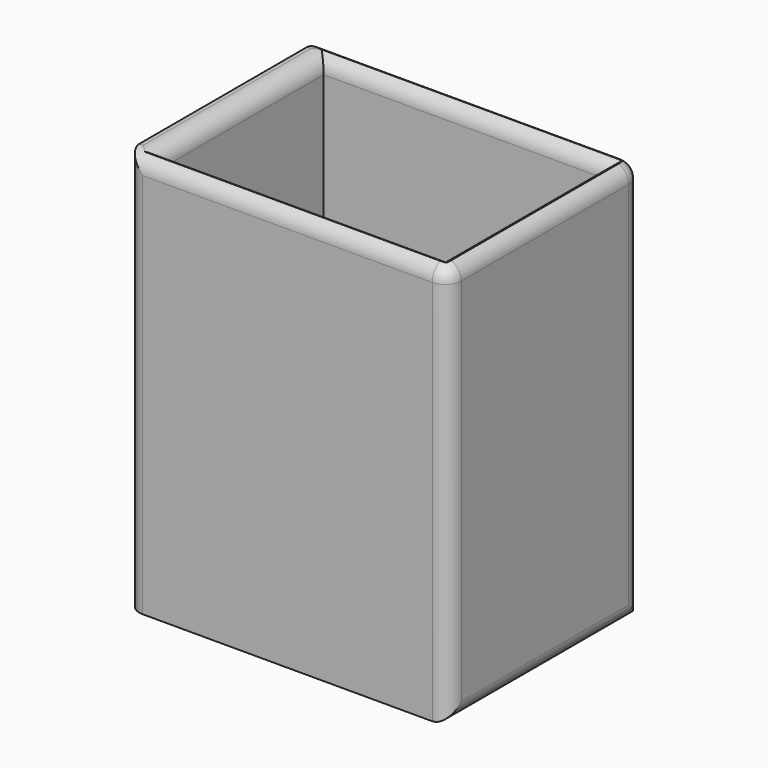
from build123d import *

# Parameters (mm, degrees)
F0_W         = 101.6
F0_H         = 76.2
F1_DEPTH     = 127
F2_T         = -6.35
F3_T1_DEPTH  = 152.4
F3_T3_DEPTH  = 134.62
F3_T5_DEPTH  = 101.6
F3_T7_DEPTH  = 66.04
F3_T9_DEPTH  = 109.22
F3_T11_DEPTH = 88.9
F3_T13_DEPTH = 63.5
F3_S17_W     = 5.1816
F3_S17_H     = 5.1816
F3_T18_DEPTH = 5.1816
F3_S23_W     = 5.1816
F3_S23_H     = 5.1816
F3_T24_DEPTH = 5.1816
F3_T31_DEPTH = 101.6
F3_T36_DEPTH = 76.2
F3_T44_DEPTH = 76.2
F3_T49_DEPTH = 101.6
F3_T57_DEPTH = 101.6
F3_T62_DEPTH = 76.2
F3_T70_DEPTH = 101.6
F3_T75_DEPTH = 76.2


# Not quite as in the source:
# - a fillet or chamfer that OpenCascade refuses, or shapes differently, is made with other operations: its cross-section is extruded or revolved along the edge and cut away or added


with BuildPart() as f1:
    # F0 (on Top) → F1 (new body)
    with BuildSketch(Plane.XY):
        with Locations((74.7453766656, -13.2239237391)):
            Rectangle(F0_W, F0_H)
    extrude(amount=F1_DEPTH)

    # F2
    f2_openings = [f1.faces().sort_by_distance(p)[0] for p in [
        (74.745377, -13.223924, 127),
    ]]
    offset(amount=F2_T, openings=f2_openings)

    # F3: fillet of radius 5.08 on 12 edges, made by hand

    # F3_s2 → F3_t1 (cut)
    with BuildSketch(Plane.XY.offset(-12.7)):
        with BuildLine():
            ThreePointArc((29.0253766656, 24.8760762609), (25.4332742171, 23.3881787093), (23.9453766656, 19.7960762609))
            Line((23.9453766656, 19.7960762609), (23.9453766656, 24.8760762609))
            Line((23.9453766656, 24.8760762609), (29.0253766656, 24.8760762609))
        make_face()
        with BuildLine():
            ThreePointArc((29.0253766656, -51.3239237391), (25.4332742171, -49.8360261876), (23.9453766656, -46.2439237391))
            Line((23.9453766656, -46.2439237391), (23.9453766656, -51.3239237391))
            Line((23.9453766656, -51.3239237391), (29.0253766656, -51.3239237391))
        make_face()
    extrude(amount=F3_T1_DEPTH, mode=Mode.SUBTRACT)

    # F3_s4 → F3_t3 (cut)
    with BuildSketch(Plane.XY.offset(-12.7)):
        with BuildLine():
            ThreePointArc((125.5453766656, 19.7960762609), (124.057479114, 23.3881787093), (120.4653766656, 24.8760762609))
            Line((120.4653766656, 24.8760762609), (125.5453766656, 24.8760762609))
            Line((125.5453766656, 24.8760762609), (125.5453766656, 19.7960762609))
        make_face()
        with BuildLine():
            ThreePointArc((120.4653766656, -51.3239237391), (124.057479114, -49.8360261876), (125.5453766656, -46.2439237391))
            Line((125.5453766656, -46.2439237391), (125.5453766656, -51.3239237391))
            Line((125.5453766656, -51.3239237391), (120.4653766656, -51.3239237391))
        make_face()
    extrude(amount=F3_T3_DEPTH, mode=Mode.SUBTRACT)

    # F3_s6 → F3_t5 (cut)
    with BuildSketch(Plane.XZ.offset(-37.5760762609)):
        with BuildLine():
            ThreePointArc((125.5453766656, 5.08), (124.057479114, 1.4878975516), (120.4653766656, 0))
            Line((120.4653766656, 0), (125.5453766656, 0))
            Line((125.5453766656, 0), (125.5453766656, 5.08))
        make_face()
    extrude(amount=F3_T5_DEPTH, mode=Mode.SUBTRACT)

    # F3_s8 → F3_t7 (cut)
    with BuildSketch(Plane.XZ.offset(-19.7960762609)):
        with BuildLine():
            ThreePointArc((125.5453766656, 121.92), (124.057479114, 125.5121024484), (120.4653766656, 127))
            Line((120.4653766656, 127), (125.5453766656, 127))
            Line((125.5453766656, 127), (125.5453766656, 121.92))
        make_face()
    extrude(amount=F3_T7_DEPTH, mode=Mode.SUBTRACT)

    # F3_s10 → F3_t9 (cut)
    with BuildSketch(Plane.YZ.offset(11.2453766656)):
        with BuildLine():
            ThreePointArc((-51.3239237391, 121.92), (-49.8360261876, 125.5121024484), (-46.2439237391, 127))
            Line((-46.2439237391, 127), (-51.3239237391, 127))
            Line((-51.3239237391, 127), (-51.3239237391, 121.92))
        make_face()
        with BuildLine():
            ThreePointArc((24.8760762609, 121.92), (23.3881787093, 125.5121024484), (19.7960762609, 127))
            Line((19.7960762609, 127), (24.8760762609, 127))
            Line((24.8760762609, 127), (24.8760762609, 121.92))
        make_face()
    extrude(amount=F3_T9_DEPTH, mode=Mode.SUBTRACT)

    # F3_s12 → F3_t11 (cut)
    with BuildSketch(Plane.YZ.offset(30.2953766656)):
        with BuildLine():
            ThreePointArc((23.6060762609, 127), (20.0139738124, 125.5121024484), (18.5260762609, 121.92))
            Line((18.5260762609, 121.92), (18.5260762609, 127))
            Line((18.5260762609, 127), (23.6060762609, 127))
        make_face()
        with BuildLine():
            ThreePointArc((-50.0539237391, 127), (-46.4618212907, 125.5121024484), (-44.9739237391, 121.92))
            Line((-44.9739237391, 121.92), (-44.9739237391, 127))
            Line((-44.9739237391, 127), (-50.0539237391, 127))
        make_face()
    extrude(amount=F3_T11_DEPTH, mode=Mode.SUBTRACT)

    # F3_s14 → F3_t13 (cut)
    with BuildSketch(Plane.XZ.offset(-18.5260762609)):
        with BuildLine():
            ThreePointArc((25.2153766656, 127), (28.807479114, 125.5121024484), (30.2953766656, 121.92))
            Line((30.2953766656, 121.92), (30.2953766656, 127))
            Line((30.2953766656, 127), (25.2153766656, 127))
        make_face()
        with BuildLine():
            ThreePointArc((124.2753766656, 127), (120.6832742171, 125.5121024484), (119.1953766656, 121.92))
            Line((119.1953766656, 121.92), (119.1953766656, 127))
            Line((119.1953766656, 127), (124.2753766656, 127))
        make_face()
    extrude(amount=F3_T13_DEPTH, mode=Mode.SUBTRACT)


with BuildPart() as f3_tool16:
    # F3_s17 → F3_t18 (new body)
    with BuildSketch(Plane.YZ.offset(120.4653766656)):
        with Locations((22.3868762609, 124.5108)):
            Rectangle(F3_S17_W, F3_S17_H)
    extrude(amount=F3_T18_DEPTH)

    # F3_s19 → F3_t20 (revolve, cut)
    with BuildSketch(Plane(origin=(120.4653766656, 19.7960762609, 121.92), x_dir=(0, -0.7071067812, -0.7071067812), z_dir=(0, -0.7071067812, 0.7071067812))):
        with BuildLine():
            ThreePointArc((0, -5.08), (5.08, 0), (0, 5.08))
            Line((0, 5.08), (0, -5.08))
        make_face()
    revolve(axis=Axis((120.4653766656, 19.7960762609, 121.92), (1, 0, 0)), mode=Mode.SUBTRACT)


with BuildPart() as f1_1:
    add(f1.part)

    # F3_t15: cut F3_tool16
    add(f3_tool16.part, mode=Mode.SUBTRACT)


with BuildPart() as f3_tool22:
    # F3_s23 → F3_t24 (new body)
    with BuildSketch(Plane.XZ.offset(46.2439237391)):
        with Locations((123.0561766656, 124.5108)):
            Rectangle(F3_S23_W, F3_S23_H)
    extrude(amount=F3_T24_DEPTH)

    # F3_s25 → F3_t26 (revolve, cut)
    with BuildSketch(Plane(origin=(120.4653766656, -46.2439237391, 121.92), x_dir=(-0.7071067812, 0, -0.7071067812), z_dir=(-0.7071067812, 0, 0.7071067812))):
        with BuildLine():
            ThreePointArc((0, -5.08), (5.08, 0), (0, 5.08))
            Line((0, 5.08), (0, -5.08))
        make_face()
    revolve(axis=Axis((120.4653766656, -46.2439237391, 121.92), (0, -1, 0)), mode=Mode.SUBTRACT)


with BuildPart() as f1_2:
    add(f1_1.part)

    # F3_t21: cut F3_tool22
    add(f3_tool22.part, mode=Mode.SUBTRACT)


with BuildPart() as f3_tool29:
    # F3_s30 → F3_t31 (new body)
    with BuildSketch(Plane.YZ.offset(131.8953766656)):
        with BuildLine():
            ThreePointArc((23.6060762609, 127), (20.0139738124, 125.5121024484), (18.5260762609, 121.92))
            Line((18.5260762609, 121.92), (18.5260762609, 127))
            Line((18.5260762609, 127), (23.6060762609, 127))
        make_face()
    extrude(amount=-F3_T31_DEPTH)

    split(bisect_by=Plane.YZ.offset(125.5453766656), keep=Keep.BOTTOM)

    split(bisect_by=Plane.YZ.offset(119.1953766656), keep=Keep.TOP)


with BuildPart() as f3_tool34:
    # F3_s35 → F3_t36 (new body)
    with BuildSketch(Plane.XZ.offset(44.9739237391)):
        with BuildLine():
            ThreePointArc((124.2753766656, 127), (120.6832742171, 125.5121024484), (119.1953766656, 121.92))
            Line((119.1953766656, 121.92), (119.1953766656, 127))
            Line((119.1953766656, 127), (124.2753766656, 127))
        make_face()
    extrude(amount=-F3_T36_DEPTH)

    split(bisect_by=Plane.XZ.offset(-24.8760762609), keep=Keep.TOP)

    split(bisect_by=Plane.XZ.offset(-18.5260762609), keep=Keep.BOTTOM)


with BuildPart() as f3_tool29_1:
    add(f3_tool29.part)

    # F3_t39: intersect F3_tool34
    add(f3_tool34.part, mode=Mode.INTERSECT)


with BuildPart() as f1_3:
    add(f1_2.part)

    # F3_t27: cut F3_tool29
    add(f3_tool29_1.part, mode=Mode.SUBTRACT)


with BuildPart() as f3_tool42:
    # F3_s43 → F3_t44 (new body)
    with BuildSketch(Plane.XZ.offset(-31.2260762609)):
        with BuildLine():
            ThreePointArc((25.2153766656, 127), (28.807479114, 125.5121024484), (30.2953766656, 121.92))
            Line((30.2953766656, 121.92), (30.2953766656, 127))
            Line((30.2953766656, 127), (25.2153766656, 127))
        make_face()
    extrude(amount=F3_T44_DEPTH)

    split(bisect_by=Plane.XZ.offset(-24.8760762609), keep=Keep.TOP)

    split(bisect_by=Plane.XZ.offset(-18.5260762609), keep=Keep.BOTTOM)


with BuildPart() as f3_tool47:
    # F3_s48 → F3_t49 (new body)
    with BuildSketch(Plane.YZ.offset(119.1953766656)):
        with BuildLine():
            ThreePointArc((23.6060762609, 127), (20.0139738124, 125.5121024484), (18.5260762609, 121.92))
            Line((18.5260762609, 121.92), (18.5260762609, 127))
            Line((18.5260762609, 127), (23.6060762609, 127))
        make_face()
    extrude(amount=-F3_T49_DEPTH)

    split(bisect_by=Plane.YZ.offset(23.9453766656), keep=Keep.TOP)

    split(bisect_by=Plane.YZ.offset(30.2953766656), keep=Keep.BOTTOM)


with BuildPart() as f3_tool42_1:
    add(f3_tool42.part)

    # F3_t52: intersect F3_tool47
    add(f3_tool47.part, mode=Mode.INTERSECT)


with BuildPart() as f1_4:
    add(f1_3.part)

    # F3_t40: cut F3_tool42
    add(f3_tool42_1.part, mode=Mode.SUBTRACT)


with BuildPart() as f3_tool55:
    # F3_s56 → F3_t57 (new body)
    with BuildSketch(Plane.YZ.offset(17.5953766656)):
        with BuildLine():
            ThreePointArc((-50.0539237391, 127), (-46.4618212907, 125.5121024484), (-44.9739237391, 121.92))
            Line((-44.9739237391, 121.92), (-44.9739237391, 127))
            Line((-44.9739237391, 127), (-50.0539237391, 127))
        make_face()
    extrude(amount=F3_T57_DEPTH)

    split(bisect_by=Plane.YZ.offset(23.9453766656), keep=Keep.TOP)

    split(bisect_by=Plane.YZ.offset(30.2953766656), keep=Keep.BOTTOM)


with BuildPart() as f3_tool60:
    # F3_s61 → F3_t62 (new body)
    with BuildSketch(Plane.XZ.offset(-18.5260762609)):
        with BuildLine():
            ThreePointArc((25.2153766656, 127), (28.807479114, 125.5121024484), (30.2953766656, 121.92))
            Line((30.2953766656, 121.92), (30.2953766656, 127))
            Line((30.2953766656, 127), (25.2153766656, 127))
        make_face()
    extrude(amount=F3_T62_DEPTH)

    split(bisect_by=Plane.XZ.offset(51.3239237391), keep=Keep.BOTTOM)

    split(bisect_by=Plane.XZ.offset(44.9739237391), keep=Keep.TOP)


with BuildPart() as f3_tool55_1:
    add(f3_tool55.part)

    # F3_t65: intersect F3_tool60
    add(f3_tool60.part, mode=Mode.INTERSECT)


with BuildPart() as f1_5:
    add(f1_4.part)

    # F3_t53: cut F3_tool55
    add(f3_tool55_1.part, mode=Mode.SUBTRACT)


with BuildPart() as f3_tool68:
    # F3_s69 → F3_t70 (new body)
    with BuildSketch(Plane.YZ.offset(30.2953766656)):
        with BuildLine():
            ThreePointArc((-50.0539237391, 127), (-46.4618212907, 125.5121024484), (-44.9739237391, 121.92))
            Line((-44.9739237391, 121.92), (-44.9739237391, 127))
            Line((-44.9739237391, 127), (-50.0539237391, 127))
        make_face()
    extrude(amount=F3_T70_DEPTH)

    split(bisect_by=Plane.YZ.offset(125.5453766656), keep=Keep.BOTTOM)

    split(bisect_by=Plane.YZ.offset(119.1953766656), keep=Keep.TOP)


with BuildPart() as f3_tool73:
    # F3_s74 → F3_t75 (new body)
    with BuildSketch(Plane.XZ.offset(57.6739237391)):
        with BuildLine():
            ThreePointArc((124.2753766656, 127), (120.6832742171, 125.5121024484), (119.1953766656, 121.92))
            Line((119.1953766656, 121.92), (119.1953766656, 127))
            Line((119.1953766656, 127), (124.2753766656, 127))
        make_face()
    extrude(amount=-F3_T75_DEPTH)

    split(bisect_by=Plane.XZ.offset(51.3239237391), keep=Keep.BOTTOM)

    split(bisect_by=Plane.XZ.offset(44.9739237391), keep=Keep.TOP)


with BuildPart() as f3_tool68_1:
    add(f3_tool68.part)

    # F3_t78: intersect F3_tool73
    add(f3_tool73.part, mode=Mode.INTERSECT)


with BuildPart() as f1_6:
    add(f1_5.part)

    # F3_t66: cut F3_tool68
    add(f3_tool68_1.part, mode=Mode.SUBTRACT)


solid = f1_6.part
